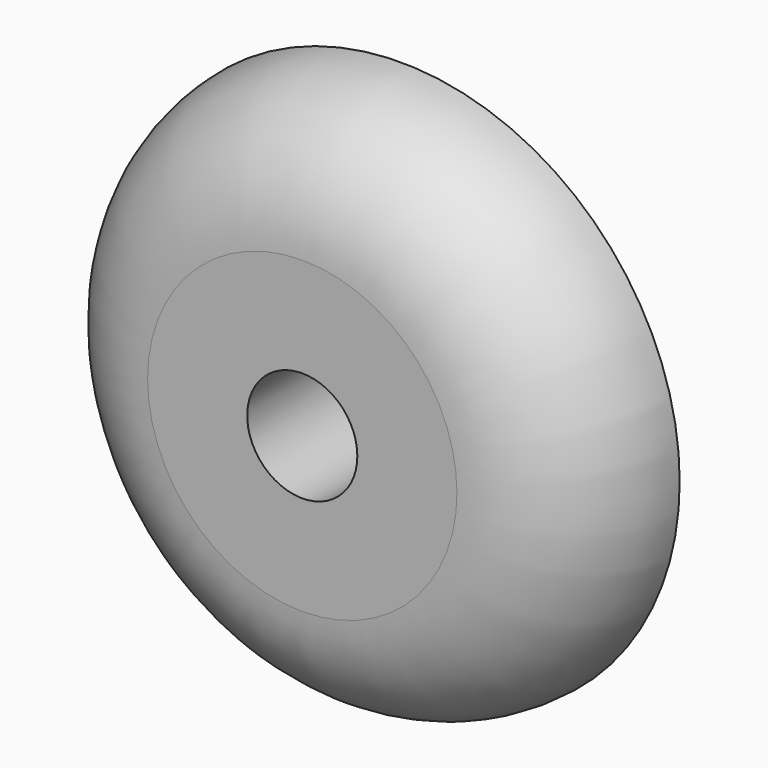
from build123d import *

# Parameters (mm, degrees)
F0_R     = 2.2225
F0_R_2   = 1.1303
F1_DEPTH = 1.27
F2_R     = 5.715
F2_R_2   = 2.2225
F2_R_3   = 1.1303
F3_DEPTH = 2.54
F4_R     = 2.53999


# Not quite as in the source:
# - a fillet or chamfer is up to 0.001 mm smaller than in the source, because OpenCascade refuses the exact size
# - a feature of the source that left no trace in its solid (it failed there, or was rolled back) is left out


with BuildPart() as f1:
    # F0 (on Front) → F1 (new body)
    with BuildSketch(Plane.XZ):
        Circle(F0_R)
        Circle(F0_R_2, mode=Mode.SUBTRACT)
    extrude(amount=F1_DEPTH)

    # F2 (on face) → F3 (join)
    with BuildSketch(Plane.XZ.offset(1.27)):
        Circle(F2_R)
        Circle(F2_R_2, mode=Mode.SUBTRACT)
        Circle(F2_R_2)
        Circle(F2_R_3, mode=Mode.SUBTRACT)
    extrude(amount=F3_DEPTH)

    # F4 (radius 2.54 in the source; OpenCascade refuses exactly that, so slightly less here)
    f4_edges = [f1.edges().sort_by_distance(p)[0] for p in [
        (-5.715, -3.81, 0),
    ]]
    fillet(f4_edges, radius=F4_R)


solid = f1.part
